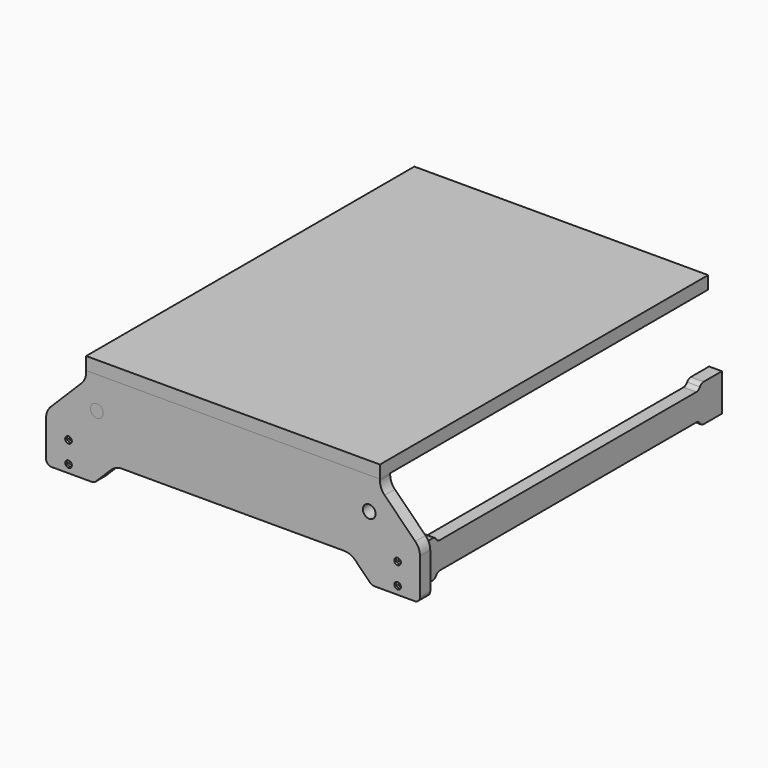
from build123d import *

# Parameters (mm, degrees)
F1_DEPTH  = 12
F2_R      = 5.975
F3_DEPTH  = 25
F4_R      = 6
F5_DEPTH  = 384
F6_W      = 275
F6_H      = 384
F7_DEPTH  = 12
F8_R      = 5
F9_R      = 15
F10_W     = 12
F10_H     = 35
F11_DEPTH = 360
F12_R     = 1
F13_DEPTH = 25
F14_R     = 3.1
F15_DEPTH = 2
F17_DEPTH = 25
F18_R     = 5


with BuildPart() as f1:
    # F0 (on Front) → F1 (new body)
    with BuildSketch(Plane.XZ):
        Polygon((137.5, 0), (-137.5, 0), (-137.5, -7.5), (-175, -45), (-175, -90), (175, -90), (175, -45), (137.5, -7.5), align=None)
    extrude(amount=F1_DEPTH)

    # F2 (on face) → F3 (cut)
    with BuildSketch(Plane.XZ.offset(12)):
        with Locations((-127.5, -30)):
            Circle(F2_R)
        with Locations((127.5, -30)):
            Circle(F2_R)
        Polygon((0, -70), (-110, -70), (-130, -90), (0, -90), (130, -90), (110, -70), align=None)
    extrude(amount=-F3_DEPTH, mode=Mode.SUBTRACT)

    # F8
    f8_edges = [f1.edges().sort_by_distance(p)[0] for p in [
        (-130, -6, -90),
        (130, -6, -90),
        (175, -6, -90),
        (-175, -6, -90),
    ]]
    fillet(f8_edges, radius=F8_R)

    # F9
    f9_edges = [f1.edges().sort_by_distance(p)[0] for p in [
        (-137.5, -6, -7.5),
        (-175, -6, -45),
        (137.5, -6, -7.5),
        (175, -6, -45),
        (-110, -6, -70),
        (110, -6, -70),
    ]]
    fillet(f9_edges, radius=F9_R)


with BuildPart() as f5:
    # F4 (on face) → F5 (new body)
    with BuildSketch(Plane.XZ.offset(12)):
        with Locations((-127.5, -30)):
            Circle(F4_R)
    extrude(amount=-F5_DEPTH)


with BuildPart() as f7:
    # F6 (on face) → F7 (new body)
    with BuildSketch(Plane.XY):
        with Locations((0, 180)):
            Rectangle(F6_W, F6_H)
    extrude(amount=F7_DEPTH)


with BuildPart() as f11:
    # F10 (on face) → F11 (new body)
    with BuildSketch(Plane(origin=(0, 0, 0), x_dir=(-1, 0, 0), z_dir=(0, 1, 0))):
        with Locations((-154, -72.5)):
            Rectangle(F10_W, F10_H)
    extrude(amount=F11_DEPTH)


with BuildPart() as f13_tool:
    # F12 (on face) → F13 (new body)
    with BuildSketch(Plane.XZ.offset(12)):
        with Locations((154, -82.5)):
            Circle(F12_R)
        with Locations((154, -62.5)):
            Circle(F12_R)
        with Locations((-154, -82.5)):
            Circle(F12_R)
        with Locations((-154, -62.5)):
            Circle(F12_R)
    extrude(amount=-F13_DEPTH)


with BuildPart() as f1_1:
    add(f1.part)

    # F13: cut by f13_tool
    add(f13_tool.part, mode=Mode.SUBTRACT)

    # F14 (on face) → F15 (cut)
    with BuildSketch(Plane.XZ.offset(12)):
        with Locations((154, -62.5)):
            Circle(F14_R)
        with Locations((154, -82.5)):
            Circle(F14_R)
        with Locations((-154, -62.5)):
            Circle(F14_R)
        with Locations((-154, -82.5)):
            Circle(F14_R)
    extrude(amount=-F15_DEPTH, mode=Mode.SUBTRACT)


with BuildPart() as f11_1:
    add(f11.part)

    # F13: cut by f13_tool
    add(f13_tool.part, mode=Mode.SUBTRACT)

    # F16 (on face) → F17 (cut)
    with BuildSketch(Plane.YZ.offset(160)):
        with BuildLine():
            Line((330.0105456627, -50), (29.9964847791, -50))
            ThreePointArc((29.9964847791, -50), (24.9964847791, -55), (29.9964847791, -60))
            Line((29.9964847791, -60), (329.9964847791, -60))
            ThreePointArc((329.9964847791, -60), (335.0035152209, -55.0070304418), (330.0105456627, -50))
        make_face()
        with BuildLine():
            ThreePointArc((330.0105456627, -95), (335.0035152209, -89.9929695582), (329.9964847791, -85))
            Line((329.9964847791, -85), (29.9964847791, -85))
            ThreePointArc((29.9964847791, -85), (24.9964847791, -90), (29.9964847791, -95))
            Line((29.9964847791, -95), (330.0105456627, -95))
        make_face()
    extrude(amount=-F17_DEPTH, mode=Mode.SUBTRACT)

    # F18
    f18_edges = [f11_1.edges().sort_by_distance(p)[0] for p in [
        (154, 24.996485, -55),
        (154, 24.996485, -90),
        (154, 335.00352, -90),
        (154, 335.00352, -55),
    ]]
    fillet(f18_edges, radius=F18_R)


solid = Compound([f5.part, f7.part, f1_1.part, f11_1.part])
